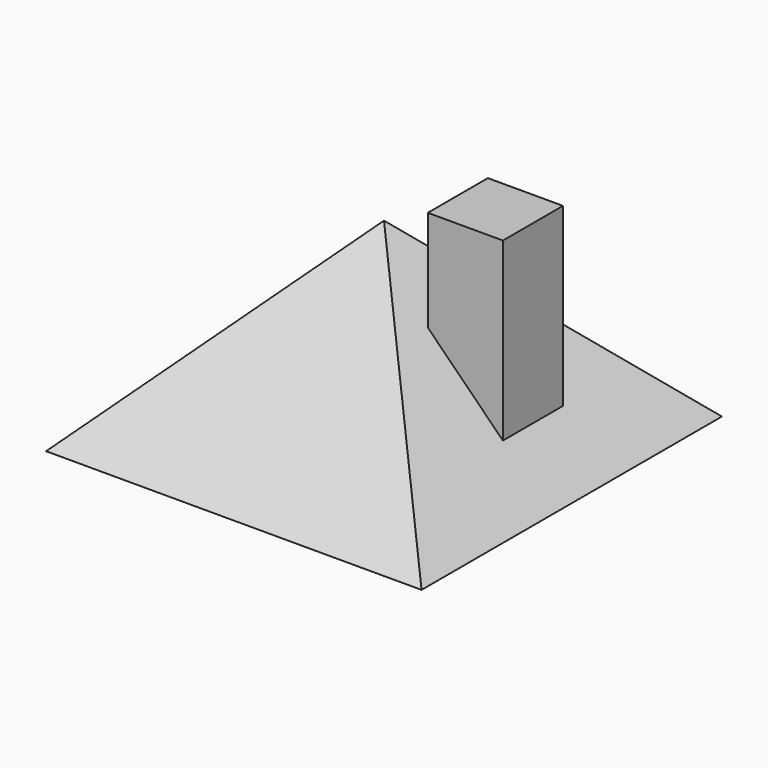
from build123d import *

# Parameters (mm, degrees)
F0_W        = 63.5
F0_H        = 63.5
F0_W_2      = 12.7
F0_H_2      = 12.7
F1_DEPTH    = 31.75
F2_T1_DEPTH = 226.8018697358
F2_T3_DEPTH = 226.8018697358
F3_DEPTH    = 38.1


# Not quite as in the source:
# - a fillet or chamfer that OpenCascade refuses, or shapes differently, is made with other operations: its cross-section is extruded or revolved along the edge and cut away or added


with BuildPart() as f1:
    # F0 (on Top) → F1 (new body)
    with BuildSketch(Plane.XY):
        with Locations((0.9875343293, -0.9437446371)):
            Rectangle(F0_W, F0_H)
        with Locations((18.0756017402, 1.2459141038)):
            Rectangle(F0_W_2, F0_H_2, mode=Mode.SUBTRACT)
    extrude(amount=F1_DEPTH)

    # F2: chamfer of 31.75 on 4 edges, made by hand

    # F2_s2 → F2_t1 (cut)
    with BuildSketch(Plane.YZ.offset(-112.4134005386)):
        Polygon((-32.6937446371, 0), (-0.9437446371, 31.75), (-32.6937446371, 31.75), align=None)
        Polygon((30.8062553629, 0), (-0.9437446371, 31.75), (30.8062553629, 31.75), align=None)
    extrude(amount=F2_T1_DEPTH, mode=Mode.SUBTRACT)

    # F2_s4 → F2_t3 (cut)
    with BuildSketch(Plane.XZ.offset(-112.4571902308)):
        Polygon((32.7375343293, 0), (0.9875343293, 31.75), (32.7375343293, 31.75), align=None)
        Polygon((-30.7624656707, 0), (0.9875343293, 31.75), (-30.7624656707, 31.75), align=None)
    extrude(amount=F2_T3_DEPTH, mode=Mode.SUBTRACT)

    # F0 (on Top) → F3 (join)
    with BuildSketch(Plane.XY):
        with Locations((18.0756017402, 1.2459141038)):
            Rectangle(F0_W_2, F0_H_2)
    extrude(amount=F3_DEPTH)


solid = f1.part
